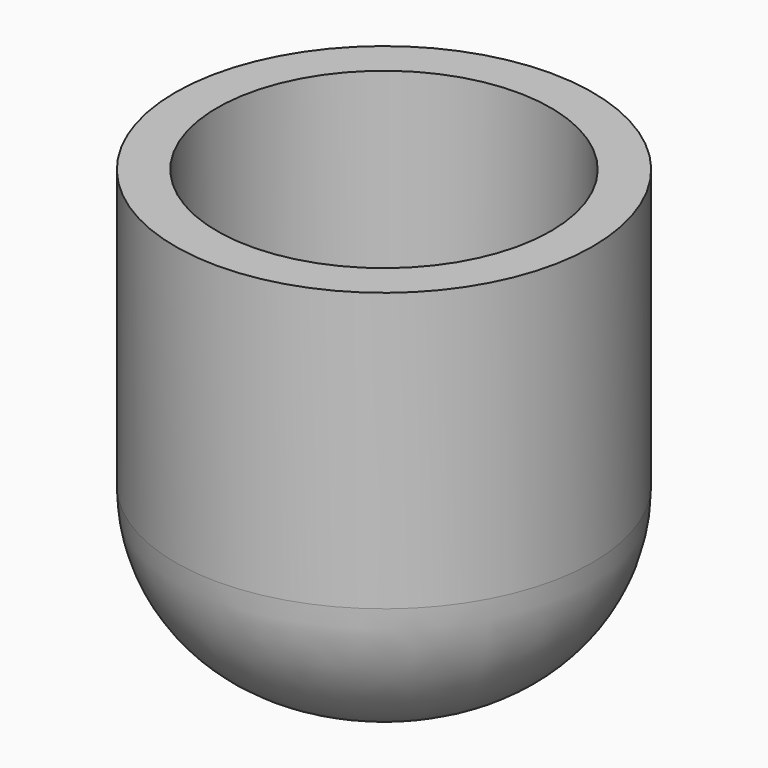
from build123d import *


# Not quite as in the source:
# - a fillet or chamfer that OpenCascade refuses, or shapes differently, is made with other operations: its cross-section is extruded or revolved along the edge and cut away or added


with BuildPart() as f1:
    # F0 (on Front) → F1 (revolve)
    with BuildSketch(Plane.XZ):
        with BuildLine():
            Line((15, 0), (13.5, 0))
            Line((13.5, 0), (12, 0))
            Line((12, 0), (12, -1.5))
            Line((12, -1.5), (12, -20))
            ThreePointArc((12, -20), (10.3452954698, -25.1406164595), (6, -28.3472333599))
            ThreePointArc((6, -28.3472333599), (5.0122671395, -28.6160728483), (4, -28.7684083747))
            Line((4, -28.7684083747), (4, -31.7684083747))
            Line((4, -31.7684083747), (6.1201079457, -31.7684083747))
            Line((6.1201079457, -31.7684083747), (6.1201079457, -31.4292851344))
            ThreePointArc((6.1201079457, -31.4292851344), (12.5191285439, -27.2367299518), (15, -20))
            Line((15, -20), (15, 0))
        make_face()
        with BuildLine():
            ThreePointArc((4, -28.7684083747), (5.0122671395, -28.6160728483), (6, -28.3472333599))
            Line((6, -28.3472333599), (6, -13.7684083747))
            Line((6, -13.7684083747), (4, -13.7684083747))
            Line((4, -13.7684083747), (4, -28.7684083747))
        make_face()
    revolve(axis=Axis((0, 0, -27.0683728158), (0, 0, -1)))

    # F2: fillet of radius 5 on 1 edges, made by hand

    # F2_s1 → F2_t2 (revolve, cut)
    with BuildSketch(Plane.XZ):
        with BuildLine():
            ThreePointArc((6, -17.7684083747), (5.472135955, -15.5323403972), (4, -13.7684083747))
            Line((4, -13.7684083747), (6, -13.7684083747))
            Line((6, -13.7684083747), (6, -17.7684083747))
        make_face()
    revolve(axis=Axis((0, 0, -13.7684083747), (0, 0, -1)), mode=Mode.SUBTRACT)


solid = f1.part
